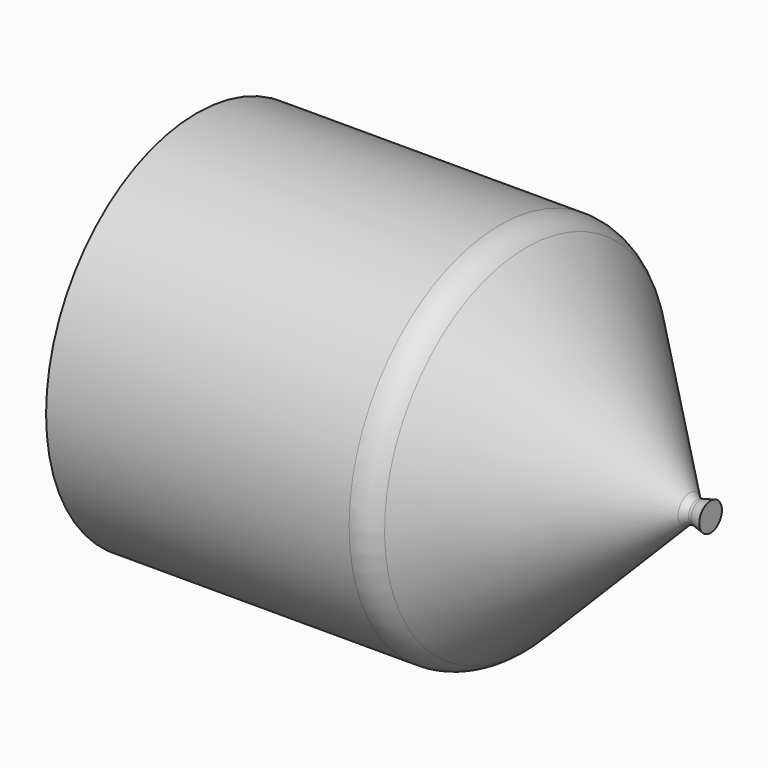
from build123d import *


# Not quite as in the source:
# - a feature of the source that left no trace in its solid (it failed there, or was rolled back) is left out


with BuildPart() as f2:
    # F0 (on Front) → F2 (revolve)
    with BuildSketch(Plane.XZ):
        with BuildLine():
            ThreePointArc((0.3778758058, 1.5097482936), (0.1905682406, 1.4724905024), (0, 1.46))
            ThreePointArc((0, 1.46), (-0.5587178113, 1.5711358825), (-1.0323759005, 1.8876240995))
            Line((-1.0323759005, 1.8876240995), (-22.680285707, 23.5355339059))
            ThreePointArc((-22.680285707, 23.5355339059), (-24.3024024511, 24.6193976626), (-26.2158196129, 25))
            Line((-26.2158196129, 25), (-66.445, 25))
            Line((-66.445, 25), (-66.445, 0))
            Line((-66.445, 0), (0, 0))
            Line((0, 0), (1.77, 0))
            Line((1.77, 0), (1.77, 1.8827668472))
            Line((1.77, 1.8827668472), (0.3778758058, 1.5097482936))
        make_face()
    revolve(axis=Axis((-33.2225, 0, 0), (-1, 0, 0)))


solid = f2.part
